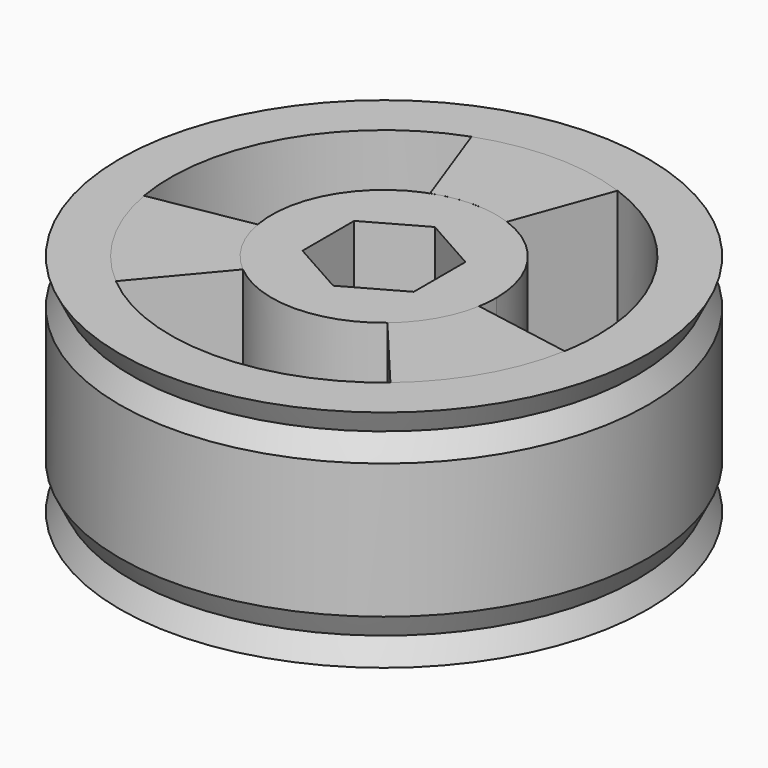
from build123d import *

# Parameters (mm, degrees)
F0_R     = 29.845
F0_R_2   = 28.575
F1_DEPTH = 5.08
F4_DEPTH = 25.4
F5_DEPTH = 20.32
F7_DEPTH = 25.4
F0_R_3   = 2.032
F8_DEPTH = 5.08


# Not quite as in the source:
# - a feature names something its author has since deleted; it is built from what else it names


with BuildPart() as f1:
    # F0 (on Top) → F1 (new body)
    with BuildSketch(Plane.XY):
        Circle(F0_R)
        Circle(F0_R_2, mode=Mode.SUBTRACT)
        Circle(F0_R_2)
        with BuildLine():
            ThreePointArc((8.2529460584, 22.6747829396), (19.7661388287, 13.8403994092), (24.13, 0))
            ThreePointArc((24.13, 0), (24.038178065, -2.1030680725), (23.7634110802, -4.1901305271))
            ThreePointArc((23.7634110802, -4.1901305271), (20.8971929933, -12.065), (15.5104650217, -18.4846524125))
            ThreePointArc((15.5104650217, -18.4846524125), (0, -24.13), (-15.5104650217, -18.4846524125))
            ThreePointArc((-15.5104650217, -18.4846524125), (-20.8971929933, -12.065), (-23.7634110802, -4.1901305271))
            ThreePointArc((-23.7634110802, -4.1901305271), (-20.8971929933, 12.065), (-8.2529460584, 22.6747829396))
            ThreePointArc((-8.2529460584, 22.6747829396), (0, 24.13), (8.2529460584, 22.6747829396))
        make_face(mode=Mode.SUBTRACT)
    extrude(amount=F1_DEPTH)

    # F2 (on Front) → F3 (revolve, cut)
    with BuildSketch(Plane.XZ):
        Polygon((-28.575, 2.54), (-29.845, 5.08), (-29.845, 0), align=None)
        Polygon((-28.575, 22.86), (-29.845, 25.4), (-29.845, 20.32), align=None)
    revolve(axis=Axis((0, 0, 0.2129347995), (0, 0, -1)), mode=Mode.SUBTRACT)


with BuildPart() as f4:
    # F0 (on Top) → F4 (new body)
    with BuildSketch(Plane.XY):
        with BuildLine():
            Line((-12.5070584633, -2.2053318564), (-23.7634110802, -4.1901305271))
            ThreePointArc((-23.7634110802, -4.1901305271), (-20.8971929933, -12.065), (-15.5104650217, -18.4846524125))
            Line((-15.5104650217, -18.4846524125), (-8.163402643, -9.7287644276))
            ThreePointArc((-8.163402643, -9.7287644276), (-10.9985226281, -6.35), (-12.5070584633, -2.2053318564))
        make_face()
    extrude(amount=F4_DEPTH)


with BuildPart() as f4b:
    # F0 (on Top) → F4, piece 2 (new body)
    with BuildSketch(Plane.XY):
        with BuildLine():
            Line((4.3436558202, 11.934096284), (8.2529460584, 22.6747829396))
            ThreePointArc((8.2529460584, 22.6747829396), (0, 24.13), (-8.2529460584, 22.6747829396))
            Line((-8.2529460584, 22.6747829396), (-4.3436558202, 11.934096284))
            ThreePointArc((-4.3436558202, 11.934096284), (0, 12.7), (4.3436558202, 11.934096284))
        make_face()
    extrude(amount=F4_DEPTH)


with BuildPart() as f4c:
    # F0 (on Top) → F4, piece 3 (new body)
    with BuildSketch(Plane.XY):
        with BuildLine():
            ThreePointArc((15.5104650217, -18.4846524125), (20.8971929933, -12.065), (23.7634110802, -4.1901305271))
            Line((23.7634110802, -4.1901305271), (12.5070584633, -2.2053318564))
            ThreePointArc((12.5070584633, -2.2053318564), (10.9985226281, -6.35), (8.163402643, -9.7287644276))
            Line((8.163402643, -9.7287644276), (15.5104650217, -18.4846524125))
        make_face()
    extrude(amount=F4_DEPTH)


with BuildPart() as f5:
    # F5 (new, through all): a face of the model
    f5_faces = [f1.part.faces().sort_by_distance(p)[0] for p in [
        (29.0008559246, 0, 5.08),
    ]]
    extrude(f5_faces, amount=F5_DEPTH)

    # F2 (on Front) → F6 (revolve, cut)
    with BuildSketch(Plane.XZ):
        Polygon((-28.575, 22.86), (-29.845, 25.4), (-29.845, 20.32), align=None)
    revolve(axis=Axis((0, 0, 0.2129347995), (0, 0, -1)), mode=Mode.SUBTRACT)


with BuildPart() as f7:
    # F0 (on Top) → F7 (new body)
    with BuildSketch(Plane.XY):
        with BuildLine():
            ThreePointArc((12.7, 0), (10.4032309625, 7.2844207417), (4.3436558202, 11.934096284))
            ThreePointArc((4.3436558202, 11.934096284), (0, 12.7), (-4.3436558202, 11.934096284))
            ThreePointArc((-4.3436558202, 11.934096284), (-10.9985226281, 6.35), (-12.5070584633, -2.2053318564))
            ThreePointArc((-12.5070584633, -2.2053318564), (-10.9985226281, -6.35), (-8.163402643, -9.7287644276))
            ThreePointArc((-8.163402643, -9.7287644276), (0, -12.7), (8.163402643, -9.7287644276))
            ThreePointArc((8.163402643, -9.7287644276), (10.9985226281, -6.35), (12.5070584633, -2.2053318564))
            ThreePointArc((12.5070584633, -2.2053318564), (12.6516726658, -1.1068779329), (12.7, 0))
        make_face()
        Polygon((0, 7.1812582227), (6.2865, 3.6409661174), (6.2865, 0), (6.2865, -3.6539388334), (0, -7.1809962018), (-6.2865, -3.6539388334), (-6.2865, 0), (-6.2865, 3.6409661174), align=None, mode=Mode.SUBTRACT)
    extrude(amount=F7_DEPTH)


with BuildPart() as f8:
    # F0 (on Top) → F8 (new body)
    with BuildSketch(Plane.XY):
        Polygon((6.2865, 0), (6.2865, 3.6409661174), (0, 7.1812582227), (-6.2865, 3.6409661174), (-6.2865, 0), (-6.2865, -3.6539388334), (0, -7.1809962018), (6.2865, -3.6539388334), align=None)
        Circle(F0_R_3, mode=Mode.SUBTRACT)
    extrude(amount=F8_DEPTH)


with BuildPart() as f8_1:
    # F9: moved
    add(f8.part.moved(Location((0, 0, 5.08))))


solid = Compound([f1.part, f4.part, f4b.part, f4c.part, f5.part, f7.part, f8_1.part])
